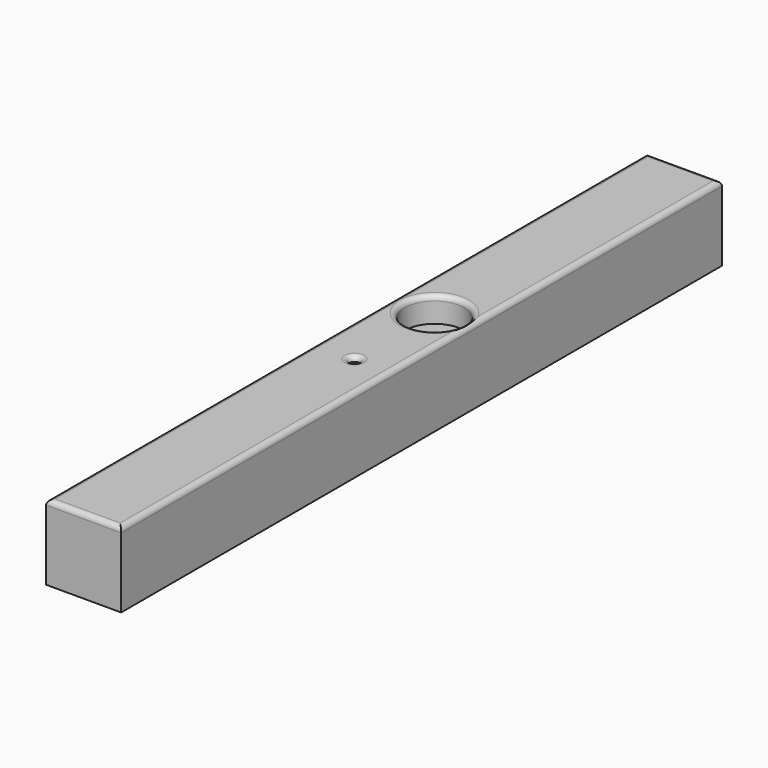
from build123d import *

# Parameters (mm, degrees)
F0_W           = 76.2
F0_H           = 76.2
F1_DEPTH       = 762
F3_D           = 5.5
F3_CBORE_D     = 9.75
F3_CBORE_DEPTH = 5
F4_R           = 30.0187668276
F5_DEPTH       = 25.4
F6_T1_DEPTH    = 787.4
F6_T3_DEPTH    = 101.6


# Not quite as in the source:
# - a fillet or chamfer that OpenCascade refuses, or shapes differently, is made with other operations: its cross-section is extruded or revolved along the edge and cut away or added


with BuildPart() as f1:
    # F0 (on Front) → F1 (new body)
    with BuildSketch(Plane.XZ):
        with Locations((-2.2192886099, 13.3160627689)):
            Rectangle(F0_W, F0_H)
    extrude(amount=F1_DEPTH)

    # F3 (through all)
    with Locations(Plane.XY.offset(51.4160627689)):
        with Locations((0, -421.1068451405)):
            CounterBoreHole(F3_D / 2, F3_CBORE_D / 2, F3_CBORE_DEPTH)

    # F4 (on face) → F5 (cut)
    with BuildSketch(Plane.XY.offset(51.4160627689)):
        with Locations((0, -319.6821808815)):
            Circle(F4_R)
    extrude(amount=-F5_DEPTH, mode=Mode.SUBTRACT)

    # F6: fillet of radius 5.08 on 6 edges, made by hand

    # F6_s2 → F6_t1 (cut)
    with BuildSketch(Plane.XZ.offset(-12.7)):
        with BuildLine():
            ThreePointArc((30.8007113901, 51.4160627689), (34.3928138385, 49.9281652174), (35.8807113901, 46.3360627689))
            Line((35.8807113901, 46.3360627689), (35.8807113901, 51.4160627689))
            Line((35.8807113901, 51.4160627689), (30.8007113901, 51.4160627689))
        make_face()
        with BuildLine():
            ThreePointArc((-35.2392886099, 51.4160627689), (-38.8313910583, 49.9281652174), (-40.3192886099, 46.3360627689))
            Line((-40.3192886099, 46.3360627689), (-40.3192886099, 51.4160627689))
            Line((-40.3192886099, 51.4160627689), (-35.2392886099, 51.4160627689))
        make_face()
    extrude(amount=F6_T1_DEPTH, mode=Mode.SUBTRACT)

    # F6_s4 → F6_t3 (cut)
    with BuildSketch(Plane.YZ.offset(-53.0192886099)):
        with BuildLine():
            ThreePointArc((-5.08, 51.4160627689), (-1.4878975516, 49.9281652174), (0, 46.3360627689))
            Line((0, 46.3360627689), (0, 51.4160627689))
            Line((0, 51.4160627689), (-5.08, 51.4160627689))
        make_face()
        with BuildLine():
            ThreePointArc((-756.92, 51.4160627689), (-760.5121024484, 49.9281652174), (-762, 46.3360627689))
            Line((-762, 46.3360627689), (-762, 51.4160627689))
            Line((-762, 51.4160627689), (-756.92, 51.4160627689))
        make_face()
    extrude(amount=F6_T3_DEPTH, mode=Mode.SUBTRACT)


with BuildPart() as f6_tool6:
    # F6_s7 → F6_t8 (revolve)
    with BuildSketch(Plane.XZ.offset(421.1068451405)):
        with BuildLine():
            ThreePointArc((9.955, 51.4160627689), (6.3628975516, 49.9281652174), (4.875, 46.3360627689))
            Line((4.875, 46.3360627689), (4.875, 51.4160627689))
            Line((4.875, 51.4160627689), (9.955, 51.4160627689))
        make_face()
    revolve(axis=Axis((0, -421.1068451405, 51.4160627689), (0, 0, 1)))

    split(bisect_by=Plane.XY.offset(46.4160627689), keep=Keep.TOP)


with BuildPart() as f1_1:
    add(f1.part)

    # F6_t5: cut F6_tool6
    add(f6_tool6.part, mode=Mode.SUBTRACT)

    # F6_s10 → F6_t11 (revolve, cut)
    with BuildSketch(Plane.XZ.offset(319.6821808815)):
        with BuildLine():
            ThreePointArc((35.0987668276, 51.4160627689), (31.5066643792, 49.9281652174), (30.0187668276, 46.3360627689))
            Line((30.0187668276, 46.3360627689), (30.0187668276, 51.4160627689))
            Line((30.0187668276, 51.4160627689), (35.0987668276, 51.4160627689))
        make_face()
    revolve(axis=Axis((0, -319.6821808815, 51.4160627689), (0, 0, 1)), mode=Mode.SUBTRACT)


solid = f1_1.part
